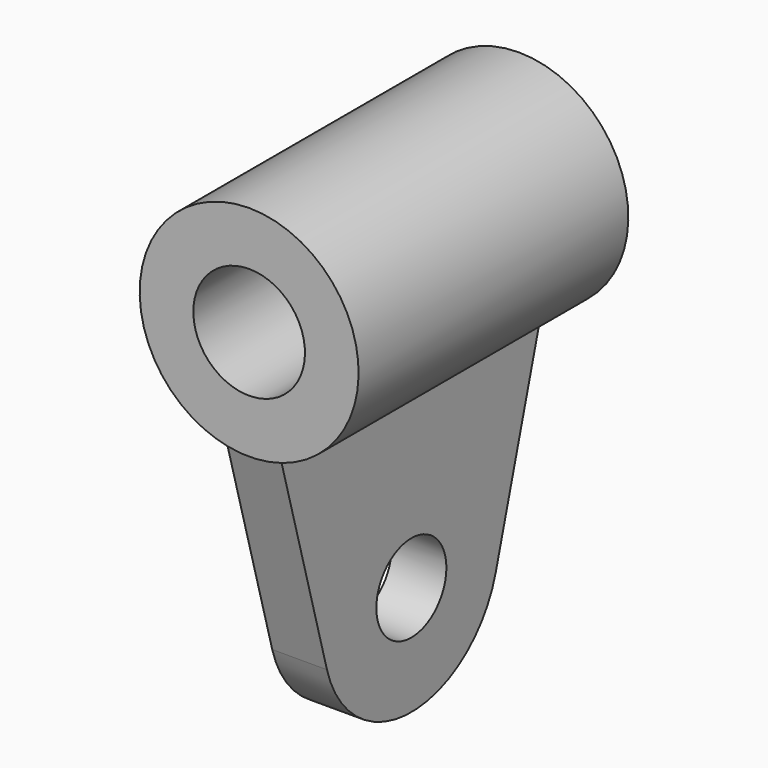
from build123d import *

# Parameters (mm, degrees)
F0_R     = 20
F1_DEPTH = 12.5
F0_W     = 154
F0_H     = 24.5


# Not quite as in the source:
# - ends of sketch curves that miss each other by under 0.0002 mm in the source are joined


with BuildPart() as f1:
    # F0 (on Right) → F1 (new body, symmetric)
    with BuildSketch(Plane.YZ):
        with BuildLine():
            Line((73.9999998675, 80), (-73.9999998675, 80))
            Line((-73.9999998675, 80), (-48.191225, -13.326883))
            ThreePointArc((-48.191225, -13.326883), (0, -50), (48.1912252169, -13.32688306))
            Line((48.1912252169, -13.32688306), (73.9999998675, 80))
        make_face()
        Circle(F0_R, mode=Mode.SUBTRACT)
        Polygon((-77, 104.5), (-77, 90.848274), (-73.9999998675, 80), (73.9999998675, 80), (77, 90.848274), (77, 104.5), align=None)
    extrude(amount=F1_DEPTH, both=True)

    # F0 (on Right) → F2 (revolve)
    with BuildSketch(Plane.YZ):
        with Locations((0, 167.75)):
            Rectangle(F0_W, F0_H)
    revolve(axis=Axis((0, 0, 130), (0, 1, 0)))


solid = f1.part
